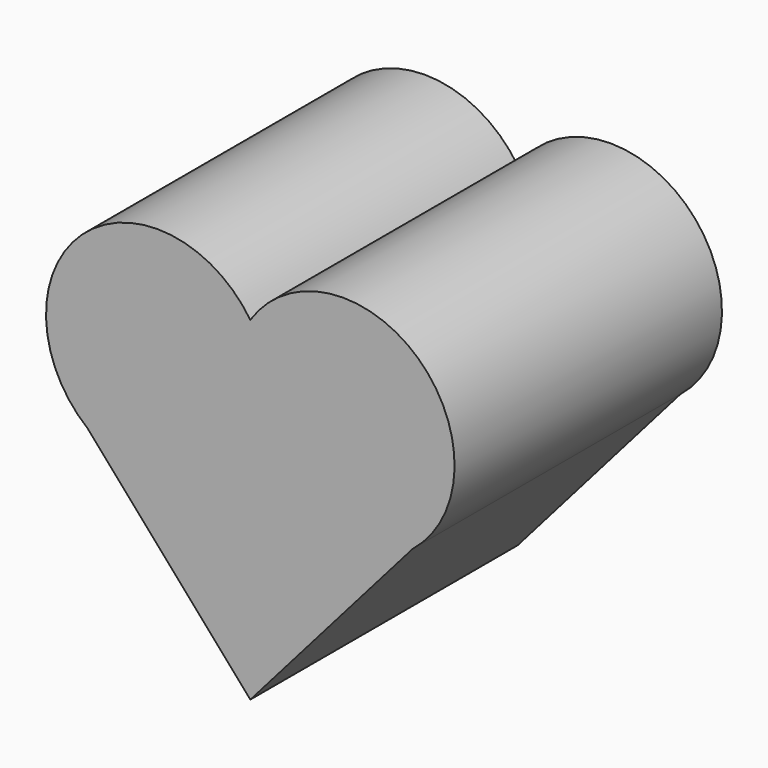
from build123d import *

# Parameters (mm, degrees)
F0_TEXT_SIZE = 7.0555555556
F1_DEPTH     = 20.32
F2_DEPTH     = 2.54


# Not quite as in the source:
# - Text() gives the source's letters only with a copy of the font that has no kerning and outlines rounded to 1/6400 em; it was checked with that copy


with BuildPart() as f1:
    # F0 (on Front) → F1 (new body)
    with BuildSketch(Plane.XZ):
        with BuildLine():
            ThreePointArc((0, 10.16), (-11.4915920882, 11.5718024828), (-11.1130920619, 0))
            Line((-11.1130920619, 0), (0, -12.7))
            Line((0, -12.7), (11.1130920619, 0))
            ThreePointArc((11.1130920619, 0), (11.4915920882, 11.5718024828), (0, 10.16))
        make_face()
        with BuildLine():
            Line((1.2477184257, -0.7813731601), (0.7549319673, -0.7813731601))
            Line((0.7549319673, -0.7813731601), (0.4936559257, -2.2487082295))
            Line((0.4936559257, -2.2487082295), (1.2477184257, -2.3424148267))
            Line((1.2477184257, -2.3424148267), (1.2102357868, -2.5937689934))
            Line((1.2102357868, -2.5937689934), (-1.1225072688, -2.5937689934))
            Line((-1.1225072688, -2.5937689934), (-1.0850246299, -2.3424148267))
            Line((-1.0850246299, -2.3424148267), (-0.5260923382, -2.2487082295))
            Line((-0.5260923382, -2.2487082295), (0.1695413423, 1.6847639927))
            Line((0.1695413423, 1.6847639927), (-0.4092346993, 1.7751632983))
            Line((-0.4092346993, 1.7751632983), (-0.3684447688, 2.0265174649))
            Line((-0.3684447688, 2.0265174649), (1.4615899534, 2.0265174649))
            add(Edge.make_bspline(
                [(1.4615899534, 2.0265174649), (2.335817384, 2.0265174649), (2.7856090507, 1.7161832636)],
                knots=[0, 0, 0, 1, 1, 1], degree=2))
            add(Edge.make_bspline(
                [(2.7856090507, 1.7161832636), (3.2354007173, 1.4058490622), (3.2354007173, 0.7928976733)],
                knots=[0, 0, 0, 1, 1, 1], degree=2))
            add(Edge.make_bspline(
                [(3.2354007173, 0.7928976733), (3.2354007173, 0.0454497566), (2.7222192937, -0.3679617017)],
                knots=[0, 0, 0, 1, 1, 1], degree=2))
            add(Edge.make_bspline(
                [(2.7222192937, -0.3679617017), (2.2090378701, -0.7813731601), (1.2477184257, -0.7813731601)],
                knots=[0, 0, 0, 1, 1, 1], degree=2))
        make_face(mode=Mode.SUBTRACT)
        with BuildLine():
            Line((6.3963501079, -0.7509480157), (5.9035636496, -0.7509480157))
            Line((5.9035636496, -0.7509480157), (5.6422876079, -2.2182830851))
            Line((5.6422876079, -2.2182830851), (6.3963501079, -2.3119896824))
            Line((6.3963501079, -2.3119896824), (6.358867469, -2.563343849))
            Line((6.358867469, -2.563343849), (4.0261244135, -2.563343849))
            Line((4.0261244135, -2.563343849), (4.0636070524, -2.3119896824))
            Line((4.0636070524, -2.3119896824), (4.622539344, -2.2182830851))
            Line((4.622539344, -2.2182830851), (5.3181730246, 1.7151891371))
            Line((5.3181730246, 1.7151891371), (4.7393969829, 1.8055884426))
            Line((4.7393969829, 1.8055884426), (4.7801869135, 2.0569426093))
            Line((4.7801869135, 2.0569426093), (6.6102216357, 2.0569426093))
            add(Edge.make_bspline(
                [(6.6102216357, 2.0569426093), (7.4844490663, 2.0569426093), (7.9342407329, 1.7466084079)],
                knots=[0, 0, 0, 1, 1, 1], degree=2))
            add(Edge.make_bspline(
                [(7.9342407329, 1.7466084079), (8.3840323996, 1.4362742065), (8.3840323996, 0.8233228176)],
                knots=[0, 0, 0, 1, 1, 1], degree=2))
            add(Edge.make_bspline(
                [(8.3840323996, 0.8233228176), (8.3840323996, 0.075874901), (7.870850976, -0.3375365574)],
                knots=[0, 0, 0, 1, 1, 1], degree=2))
            add(Edge.make_bspline(
                [(7.870850976, -0.3375365574), (7.3576695524, -0.7509480157), (6.3963501079, -0.7509480157)],
                knots=[0, 0, 0, 1, 1, 1], degree=2))
        make_face(mode=Mode.SUBTRACT)
        with BuildLine():
            Line((-7.8795292713, 5.9941915975), (-9.1296855213, 5.9941915975))
            Line((-9.1296855213, 5.9941915975), (-9.4295466324, 4.2997558336))
            Line((-9.4295466324, 4.2997558336), (-8.678791424, 4.2060492364))
            Line((-8.678791424, 4.2060492364), (-8.7206837851, 3.9546950698))
            Line((-8.7206837851, 3.9546950698), (-11.0523244101, 3.9546950698))
            Line((-11.0523244101, 3.9546950698), (-11.0115344796, 4.2060492364))
            Line((-11.0115344796, 4.2060492364), (-10.4459876046, 4.2997558336))
            Line((-10.4459876046, 4.2997558336), (-9.7536612157, 8.2332280559))
            Line((-9.7536612157, 8.2332280559), (-10.3291299657, 8.3236273614))
            Line((-10.3291299657, 8.3236273614), (-10.2839303129, 8.5749815281))
            Line((-10.2839303129, 8.5749815281), (-6.456291424, 8.5749815281))
            Line((-6.456291424, 8.5749815281), (-6.6767775351, 7.3314398614))
            Line((-6.6767775351, 7.3314398614), (-7.0008921185, 7.3314398614))
            Line((-7.0008921185, 7.3314398614), (-6.9667167713, 8.1472384725))
            add(Edge.make_bspline(
                [(-6.9667167713, 8.1472384725), (-7.1353886463, 8.1714919448), (-7.5747072226, 8.1836186809)],
                knots=[0, 0, 0, 1, 1, 1], degree=2))
            add(Edge.make_bspline(
                [(-7.5747072226, 8.1836186809), (-8.014025799, 8.195745417), (-8.2653799657, 8.195745417)],
                knots=[0, 0, 0, 1, 1, 1], degree=2))
            Line((-8.2653799657, 8.195745417), (-8.7405275351, 8.195745417))
            Line((-8.7405275351, 8.195745417), (-9.0613348268, 6.3734277086))
            Line((-9.0613348268, 6.3734277086), (-7.8111785768, 6.3734277086))
            Line((-7.8111785768, 6.3734277086), (-7.6006143407, 6.9588183336))
            Line((-7.6006143407, 6.9588183336), (-7.2941386463, 6.9588183336))
            Line((-7.2941386463, 6.9588183336), (-7.5697462851, 5.4021863892))
            Line((-7.5697462851, 5.4021863892), (-7.8762219796, 5.4021863892))
            Line((-7.8762219796, 5.4021863892), (-7.8795292713, 5.9941915975))
        make_face(mode=Mode.SUBTRACT)
        with BuildLine():
            Line((-2.3126734355, 5.973310882), (-3.5628296855, 5.973310882))
            Line((-3.5628296855, 5.973310882), (-3.8626907966, 4.2788751181))
            Line((-3.8626907966, 4.2788751181), (-3.1119355883, 4.1851685209))
            Line((-3.1119355883, 4.1851685209), (-3.1538279494, 3.9338143542))
            Line((-3.1538279494, 3.9338143542), (-5.4854685744, 3.9338143542))
            Line((-5.4854685744, 3.9338143542), (-5.4446786438, 4.1851685209))
            Line((-5.4446786438, 4.1851685209), (-4.8791317688, 4.2788751181))
            Line((-4.8791317688, 4.2788751181), (-4.1868053799, 8.2123473404))
            Line((-4.1868053799, 8.2123473404), (-4.7622741299, 8.3027466459))
            Line((-4.7622741299, 8.3027466459), (-4.7170744772, 8.5541008126))
            Line((-4.7170744772, 8.5541008126), (-0.8894355883, 8.5541008126))
            Line((-0.8894355883, 8.5541008126), (-1.1099216994, 7.3105591459))
            Line((-1.1099216994, 7.3105591459), (-1.4340362827, 7.3105591459))
            Line((-1.4340362827, 7.3105591459), (-1.3998609355, 8.126357757))
            add(Edge.make_bspline(
                [(-1.3998609355, 8.126357757), (-1.5685328105, 8.1506112292), (-2.0078513869, 8.1627379654)],
                knots=[0, 0, 0, 1, 1, 1], degree=2))
            add(Edge.make_bspline(
                [(-2.0078513869, 8.1627379654), (-2.4471699633, 8.1748647015), (-2.6985241299, 8.1748647015)],
                knots=[0, 0, 0, 1, 1, 1], degree=2))
            Line((-2.6985241299, 8.1748647015), (-3.1736716994, 8.1748647015))
            Line((-3.1736716994, 8.1748647015), (-3.4944789911, 6.3525469931))
            Line((-3.4944789911, 6.3525469931), (-2.2443227411, 6.3525469931))
            Line((-2.2443227411, 6.3525469931), (-2.0337585049, 6.9379376181))
            Line((-2.0337585049, 6.9379376181), (-1.7272828105, 6.9379376181))
            Line((-1.7272828105, 6.9379376181), (-2.0028904494, 5.3813056737))
            Line((-2.0028904494, 5.3813056737), (-2.3093661438, 5.3813056737))
            Line((-2.3093661438, 5.3813056737), (-2.3126734355, 5.973310882))
        make_face(mode=Mode.SUBTRACT)
        with Locations((-11.0457098268, 3.9546950698)):
            Text('F', F0_TEXT_SIZE, font='Tinos', font_style=FontStyle.BOLDITALIC, text_align=(TextAlign.LEFT, TextAlign.BOTTOM))
        with Locations((-5.4788539911, 3.9338143542)):
            Text('F', F0_TEXT_SIZE, font='Tinos', font_style=FontStyle.BOLDITALIC, text_align=(TextAlign.LEFT, TextAlign.BOTTOM))
        with Locations((4.0294317051, -2.563343849)):
            Text('P', F0_TEXT_SIZE, font='Tinos', font_style=FontStyle.BOLDITALIC, text_align=(TextAlign.LEFT, TextAlign.BOTTOM))
        with BuildLine():
            Line((5.9730167746, -0.3717119046), (6.2442146913, -0.3717119046))
            add(Edge.make_bspline(
                [(6.2442146913, -0.3717119046), (6.7722789274, -0.3717119046), (7.073242469, -0.053109474)],
                knots=[0, 0, 0, 1, 1, 1], degree=2))
            add(Edge.make_bspline(
                [(7.073242469, -0.053109474), (7.3742060107, 0.2654929565), (7.3742060107, 0.8134009426)],
                knots=[0, 0, 0, 1, 1, 1], degree=2))
            add(Edge.make_bspline(
                [(7.3742060107, 0.8134009426), (7.3742060107, 1.226812401), (7.1730124343, 1.4506058037)],
                knots=[0, 0, 0, 1, 1, 1], degree=2))
            add(Edge.make_bspline(
                [(7.1730124343, 1.4506058037), (6.9718188579, 1.6743992065), (6.5716365663, 1.6743992065)],
                knots=[0, 0, 0, 1, 1, 1], degree=2))
            Line((6.5716365663, 1.6743992065), (6.3346139968, 1.6743992065))
            Line((6.3346139968, 1.6743992065), (5.9730167746, -0.3717119046))
        make_face()
        with Locations((-1.1191999771, -2.5937689934)):
            Text('P', F0_TEXT_SIZE, font='Tinos', font_style=FontStyle.BOLDITALIC, text_align=(TextAlign.LEFT, TextAlign.BOTTOM))
        with BuildLine():
            Line((0.8243850923, -0.4021370489), (1.095583009, -0.4021370489))
            add(Edge.make_bspline(
                [(1.095583009, -0.4021370489), (1.6236472451, -0.4021370489), (1.9246107868, -0.0835346184)],
                knots=[0, 0, 0, 1, 1, 1], degree=2))
            add(Edge.make_bspline(
                [(1.9246107868, -0.0835346184), (2.2255743284, 0.2350678122), (2.2255743284, 0.7829757983)],
                knots=[0, 0, 0, 1, 1, 1], degree=2))
            add(Edge.make_bspline(
                [(2.2255743284, 0.7829757983), (2.2255743284, 1.1963872566), (2.0243807521, 1.4201806594)],
                knots=[0, 0, 0, 1, 1, 1], degree=2))
            add(Edge.make_bspline(
                [(2.0243807521, 1.4201806594), (1.8231871757, 1.6439740622), (1.423004884, 1.6439740622)],
                knots=[0, 0, 0, 1, 1, 1], degree=2))
            Line((1.423004884, 1.6439740622), (1.1859823146, 1.6439740622))
            Line((1.1859823146, 1.6439740622), (0.8243850923, -0.4021370489))
        make_face()
    extrude(amount=F1_DEPTH)

    # F0 (on Front) → F2 (join)
    with BuildSketch(Plane.XZ):
        with BuildLine():
            ThreePointArc((0, 10.16), (-11.4915920882, 11.5718024828), (-11.1130920619, 0))
            Line((-11.1130920619, 0), (0, -12.7))
            Line((0, -12.7), (11.1130920619, 0))
            ThreePointArc((11.1130920619, 0), (11.4915920882, 11.5718024828), (0, 10.16))
        make_face()
        with BuildLine():
            Line((1.2477184257, -0.7813731601), (0.7549319673, -0.7813731601))
            Line((0.7549319673, -0.7813731601), (0.4936559257, -2.2487082295))
            Line((0.4936559257, -2.2487082295), (1.2477184257, -2.3424148267))
            Line((1.2477184257, -2.3424148267), (1.2102357868, -2.5937689934))
            Line((1.2102357868, -2.5937689934), (-1.1225072688, -2.5937689934))
            Line((-1.1225072688, -2.5937689934), (-1.0850246299, -2.3424148267))
            Line((-1.0850246299, -2.3424148267), (-0.5260923382, -2.2487082295))
            Line((-0.5260923382, -2.2487082295), (0.1695413423, 1.6847639927))
            Line((0.1695413423, 1.6847639927), (-0.4092346993, 1.7751632983))
            Line((-0.4092346993, 1.7751632983), (-0.3684447688, 2.0265174649))
            Line((-0.3684447688, 2.0265174649), (1.4615899534, 2.0265174649))
            add(Edge.make_bspline(
                [(1.4615899534, 2.0265174649), (2.335817384, 2.0265174649), (2.7856090507, 1.7161832636)],
                knots=[0, 0, 0, 1, 1, 1], degree=2))
            add(Edge.make_bspline(
                [(2.7856090507, 1.7161832636), (3.2354007173, 1.4058490622), (3.2354007173, 0.7928976733)],
                knots=[0, 0, 0, 1, 1, 1], degree=2))
            add(Edge.make_bspline(
                [(3.2354007173, 0.7928976733), (3.2354007173, 0.0454497566), (2.7222192937, -0.3679617017)],
                knots=[0, 0, 0, 1, 1, 1], degree=2))
            add(Edge.make_bspline(
                [(2.7222192937, -0.3679617017), (2.2090378701, -0.7813731601), (1.2477184257, -0.7813731601)],
                knots=[0, 0, 0, 1, 1, 1], degree=2))
        make_face(mode=Mode.SUBTRACT)
        with BuildLine():
            Line((6.3963501079, -0.7509480157), (5.9035636496, -0.7509480157))
            Line((5.9035636496, -0.7509480157), (5.6422876079, -2.2182830851))
            Line((5.6422876079, -2.2182830851), (6.3963501079, -2.3119896824))
            Line((6.3963501079, -2.3119896824), (6.358867469, -2.563343849))
            Line((6.358867469, -2.563343849), (4.0261244135, -2.563343849))
            Line((4.0261244135, -2.563343849), (4.0636070524, -2.3119896824))
            Line((4.0636070524, -2.3119896824), (4.622539344, -2.2182830851))
            Line((4.622539344, -2.2182830851), (5.3181730246, 1.7151891371))
            Line((5.3181730246, 1.7151891371), (4.7393969829, 1.8055884426))
            Line((4.7393969829, 1.8055884426), (4.7801869135, 2.0569426093))
            Line((4.7801869135, 2.0569426093), (6.6102216357, 2.0569426093))
            add(Edge.make_bspline(
                [(6.6102216357, 2.0569426093), (7.4844490663, 2.0569426093), (7.9342407329, 1.7466084079)],
                knots=[0, 0, 0, 1, 1, 1], degree=2))
            add(Edge.make_bspline(
                [(7.9342407329, 1.7466084079), (8.3840323996, 1.4362742065), (8.3840323996, 0.8233228176)],
                knots=[0, 0, 0, 1, 1, 1], degree=2))
            add(Edge.make_bspline(
                [(8.3840323996, 0.8233228176), (8.3840323996, 0.075874901), (7.870850976, -0.3375365574)],
                knots=[0, 0, 0, 1, 1, 1], degree=2))
            add(Edge.make_bspline(
                [(7.870850976, -0.3375365574), (7.3576695524, -0.7509480157), (6.3963501079, -0.7509480157)],
                knots=[0, 0, 0, 1, 1, 1], degree=2))
        make_face(mode=Mode.SUBTRACT)
        with BuildLine():
            Line((-7.8795292713, 5.9941915975), (-9.1296855213, 5.9941915975))
            Line((-9.1296855213, 5.9941915975), (-9.4295466324, 4.2997558336))
            Line((-9.4295466324, 4.2997558336), (-8.678791424, 4.2060492364))
            Line((-8.678791424, 4.2060492364), (-8.7206837851, 3.9546950698))
            Line((-8.7206837851, 3.9546950698), (-11.0523244101, 3.9546950698))
            Line((-11.0523244101, 3.9546950698), (-11.0115344796, 4.2060492364))
            Line((-11.0115344796, 4.2060492364), (-10.4459876046, 4.2997558336))
            Line((-10.4459876046, 4.2997558336), (-9.7536612157, 8.2332280559))
            Line((-9.7536612157, 8.2332280559), (-10.3291299657, 8.3236273614))
            Line((-10.3291299657, 8.3236273614), (-10.2839303129, 8.5749815281))
            Line((-10.2839303129, 8.5749815281), (-6.456291424, 8.5749815281))
            Line((-6.456291424, 8.5749815281), (-6.6767775351, 7.3314398614))
            Line((-6.6767775351, 7.3314398614), (-7.0008921185, 7.3314398614))
            Line((-7.0008921185, 7.3314398614), (-6.9667167713, 8.1472384725))
            add(Edge.make_bspline(
                [(-6.9667167713, 8.1472384725), (-7.1353886463, 8.1714919448), (-7.5747072226, 8.1836186809)],
                knots=[0, 0, 0, 1, 1, 1], degree=2))
            add(Edge.make_bspline(
                [(-7.5747072226, 8.1836186809), (-8.014025799, 8.195745417), (-8.2653799657, 8.195745417)],
                knots=[0, 0, 0, 1, 1, 1], degree=2))
            Line((-8.2653799657, 8.195745417), (-8.7405275351, 8.195745417))
            Line((-8.7405275351, 8.195745417), (-9.0613348268, 6.3734277086))
            Line((-9.0613348268, 6.3734277086), (-7.8111785768, 6.3734277086))
            Line((-7.8111785768, 6.3734277086), (-7.6006143407, 6.9588183336))
            Line((-7.6006143407, 6.9588183336), (-7.2941386463, 6.9588183336))
            Line((-7.2941386463, 6.9588183336), (-7.5697462851, 5.4021863892))
            Line((-7.5697462851, 5.4021863892), (-7.8762219796, 5.4021863892))
            Line((-7.8762219796, 5.4021863892), (-7.8795292713, 5.9941915975))
        make_face(mode=Mode.SUBTRACT)
        with BuildLine():
            Line((-2.3126734355, 5.973310882), (-3.5628296855, 5.973310882))
            Line((-3.5628296855, 5.973310882), (-3.8626907966, 4.2788751181))
            Line((-3.8626907966, 4.2788751181), (-3.1119355883, 4.1851685209))
            Line((-3.1119355883, 4.1851685209), (-3.1538279494, 3.9338143542))
            Line((-3.1538279494, 3.9338143542), (-5.4854685744, 3.9338143542))
            Line((-5.4854685744, 3.9338143542), (-5.4446786438, 4.1851685209))
            Line((-5.4446786438, 4.1851685209), (-4.8791317688, 4.2788751181))
            Line((-4.8791317688, 4.2788751181), (-4.1868053799, 8.2123473404))
            Line((-4.1868053799, 8.2123473404), (-4.7622741299, 8.3027466459))
            Line((-4.7622741299, 8.3027466459), (-4.7170744772, 8.5541008126))
            Line((-4.7170744772, 8.5541008126), (-0.8894355883, 8.5541008126))
            Line((-0.8894355883, 8.5541008126), (-1.1099216994, 7.3105591459))
            Line((-1.1099216994, 7.3105591459), (-1.4340362827, 7.3105591459))
            Line((-1.4340362827, 7.3105591459), (-1.3998609355, 8.126357757))
            add(Edge.make_bspline(
                [(-1.3998609355, 8.126357757), (-1.5685328105, 8.1506112292), (-2.0078513869, 8.1627379654)],
                knots=[0, 0, 0, 1, 1, 1], degree=2))
            add(Edge.make_bspline(
                [(-2.0078513869, 8.1627379654), (-2.4471699633, 8.1748647015), (-2.6985241299, 8.1748647015)],
                knots=[0, 0, 0, 1, 1, 1], degree=2))
            Line((-2.6985241299, 8.1748647015), (-3.1736716994, 8.1748647015))
            Line((-3.1736716994, 8.1748647015), (-3.4944789911, 6.3525469931))
            Line((-3.4944789911, 6.3525469931), (-2.2443227411, 6.3525469931))
            Line((-2.2443227411, 6.3525469931), (-2.0337585049, 6.9379376181))
            Line((-2.0337585049, 6.9379376181), (-1.7272828105, 6.9379376181))
            Line((-1.7272828105, 6.9379376181), (-2.0028904494, 5.3813056737))
            Line((-2.0028904494, 5.3813056737), (-2.3093661438, 5.3813056737))
            Line((-2.3093661438, 5.3813056737), (-2.3126734355, 5.973310882))
        make_face(mode=Mode.SUBTRACT)
        with BuildLine():
            Line((5.9730167746, -0.3717119046), (6.2442146913, -0.3717119046))
            add(Edge.make_bspline(
                [(6.2442146913, -0.3717119046), (6.7722789274, -0.3717119046), (7.073242469, -0.053109474)],
                knots=[0, 0, 0, 1, 1, 1], degree=2))
            add(Edge.make_bspline(
                [(7.073242469, -0.053109474), (7.3742060107, 0.2654929565), (7.3742060107, 0.8134009426)],
                knots=[0, 0, 0, 1, 1, 1], degree=2))
            add(Edge.make_bspline(
                [(7.3742060107, 0.8134009426), (7.3742060107, 1.226812401), (7.1730124343, 1.4506058037)],
                knots=[0, 0, 0, 1, 1, 1], degree=2))
            add(Edge.make_bspline(
                [(7.1730124343, 1.4506058037), (6.9718188579, 1.6743992065), (6.5716365663, 1.6743992065)],
                knots=[0, 0, 0, 1, 1, 1], degree=2))
            Line((6.5716365663, 1.6743992065), (6.3346139968, 1.6743992065))
            Line((6.3346139968, 1.6743992065), (5.9730167746, -0.3717119046))
        make_face()
        with BuildLine():
            Line((0.8243850923, -0.4021370489), (1.095583009, -0.4021370489))
            add(Edge.make_bspline(
                [(1.095583009, -0.4021370489), (1.6236472451, -0.4021370489), (1.9246107868, -0.0835346184)],
                knots=[0, 0, 0, 1, 1, 1], degree=2))
            add(Edge.make_bspline(
                [(1.9246107868, -0.0835346184), (2.2255743284, 0.2350678122), (2.2255743284, 0.7829757983)],
                knots=[0, 0, 0, 1, 1, 1], degree=2))
            add(Edge.make_bspline(
                [(2.2255743284, 0.7829757983), (2.2255743284, 1.1963872566), (2.0243807521, 1.4201806594)],
                knots=[0, 0, 0, 1, 1, 1], degree=2))
            add(Edge.make_bspline(
                [(2.0243807521, 1.4201806594), (1.8231871757, 1.6439740622), (1.423004884, 1.6439740622)],
                knots=[0, 0, 0, 1, 1, 1], degree=2))
            Line((1.423004884, 1.6439740622), (1.1859823146, 1.6439740622))
            Line((1.1859823146, 1.6439740622), (0.8243850923, -0.4021370489))
        make_face()
    extrude(amount=-F2_DEPTH)


solid = f1.part
